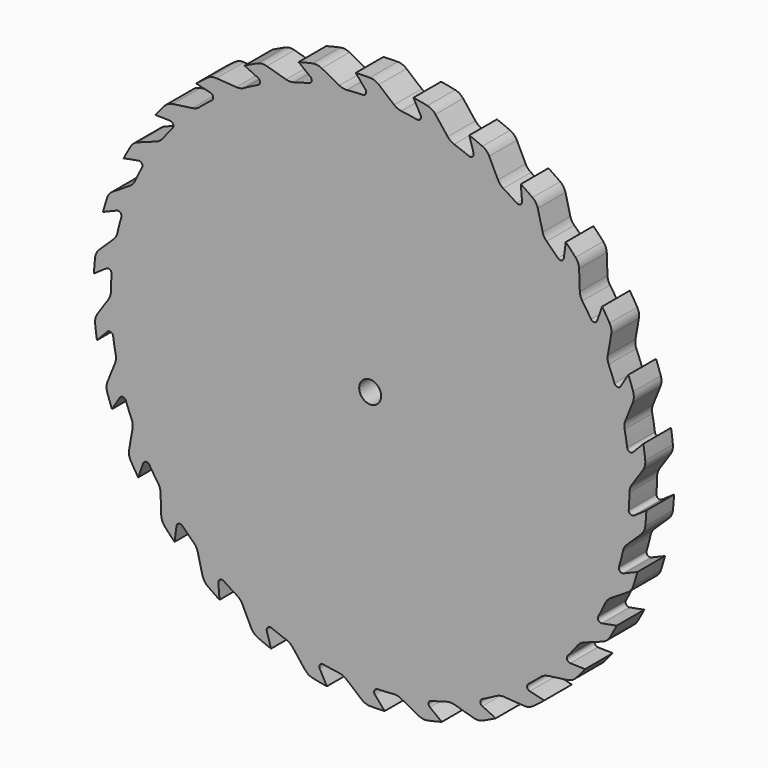
from build123d import *

# Parameters (mm, degrees)
F0_R            = 40
F1_DEPTH        = 5
F4_DEPTH        = 25
F4_COPIES_COUNT = 30
F5_R            = 2
F6_R            = 0.5
F7_R            = 1.5875
F8_DEPTH        = 25


# Not quite as in the source:
# - a pattern or mirror of a feature is missing from the dataset's text; its kind, count and spacing are read off the source's solid


with BuildPart() as f1:
    # F0 (on Front) → F1 (new body)
    with BuildSketch(Plane.XZ):
        Circle(F0_R)
    extrude(amount=F1_DEPTH)

    # F2 (on face) → F4 (cut)
    with BuildSketch(Plane.XZ.offset(5)):
        with BuildLine():
            Line((-7.6323598151, 39.2650873379), (-3.9198173725, 37.2945710763))
            ThreePointArc((-3.9198173725, 37.2945710763), (-1.9625983591, 37.4486075533), (0, 37.5))
            Line((0, 37.5), (-2.0934382497, 39.9451813902))
            ThreePointArc((-2.0934382497, 39.9451813902), (-4.8747737362, 39.7018460657), (-7.6323598151, 39.2650873379))
        make_face()
    f4 = extrude(amount=-F4_DEPTH, mode=Mode.SUBTRACT)

    # F4_copies: F4 ×30 about axis
    f4_copies_axis = Axis((0, 0, 0), (0, 1, 0))
    for i in range(1, F4_COPIES_COUNT):
        add(f4.rotate(f4_copies_axis, i * 360 / F4_COPIES_COUNT), mode=Mode.SUBTRACT)

    # F5
    f5_edges = [f1.edges().sort_by_distance(p)[0] for p in [
        (-7.63236, -2.5, 39.265087),
        (-3.919817, -2.5, 37.294571),
        (0.698096, -2.5, 39.993908),
        (3.919817, -2.5, 37.294571),
        (8.998042, -2.5, 38.974803),
        (11.588137, -2.5, 35.664619),
        (16.90473, -2.5, 36.252311),
        (18.75, -2.5, 32.475953),
        (24.072601, -2.5, 31.94542),
        (25.092398, -2.5, 27.867931),
        (30.188383, -2.5, 26.242361),
        (30.338137, -2.5, 22.041947),
        (34.984788, -2.5, 19.392385),
        (34.257955, -2.5, 15.252624),
        (38.25219, -2.5, 11.694868),
        (36.680535, -2.5, 7.796688),
        (39.847788, -2.5, 3.48623),
        (37.5, -2.5, 0),
        (39.701846, -2.5, -4.874774),
        (36.680535, -2.5, -7.796688),
        (37.820743, -2.5, -13.022726),
        (34.257955, -2.5, -15.252624),
        (34.286692, -2.5, -20.601523),
        (30.338137, -2.5, -22.041947),
        (29.254148, -2.5, -27.279934),
        (25.092398, -2.5, -27.867931),
        (22.943057, -2.5, -32.766082),
        (18.75, -2.5, -32.475953),
        (15.629245, -2.5, -36.820194),
        (11.588137, -2.5, -35.664619),
        (7.63236, -2.5, -39.265087),
        (3.919817, -2.5, -37.294571),
        (-0.698096, -2.5, -39.993908),
        (-3.919817, -2.5, -37.294571),
        (-8.998042, -2.5, -38.974803),
        (-11.588137, -2.5, -35.664619),
        (-16.90473, -2.5, -36.252311),
        (-18.75, -2.5, -32.475953),
        (-24.072601, -2.5, -31.94542),
        (-25.092398, -2.5, -27.867931),
        (-30.188383, -2.5, -26.242361),
        (-30.338137, -2.5, -22.041947),
        (-34.984788, -2.5, -19.392385),
        (-34.257955, -2.5, -15.252624),
        (-38.25219, -2.5, -11.694868),
        (-36.680535, -2.5, -7.796688),
        (-39.847788, -2.5, -3.48623),
        (-37.5, -2.5, 0),
        (-39.701846, -2.5, 4.874774),
        (-36.680535, -2.5, 7.796688),
        (-37.820743, -2.5, 13.022726),
        (-34.257955, -2.5, 15.252624),
        (-34.286692, -2.5, 20.601523),
        (-30.338137, -2.5, 22.041947),
        (-29.254148, -2.5, 27.279934),
        (-25.092398, -2.5, 27.867931),
        (-22.943057, -2.5, 32.766082),
        (-18.75, -2.5, 32.475953),
        (-15.629245, -2.5, 36.820194),
        (-11.588137, -2.5, 35.664619),
    ]]
    fillet(f5_edges, radius=F5_R)

    # F6
    f6_edges = [f1.edges().sort_by_distance(p)[0] for p in [
        (0, -2.5, 37.5),
        (-7.796688, -2.5, 36.680535),
        (7.796688, -2.5, 36.680535),
        (-15.252624, -2.5, 34.257955),
        (15.252624, -2.5, 34.257955),
        (-22.041947, -2.5, 30.338137),
        (22.041947, -2.5, 30.338137),
        (-27.867931, -2.5, 25.092398),
        (27.867931, -2.5, 25.092398),
        (-32.475953, -2.5, 18.75),
        (32.475953, -2.5, 18.75),
        (-35.664619, -2.5, 11.588137),
        (35.664619, -2.5, 11.588137),
        (-37.294571, -2.5, 3.919817),
        (37.294571, -2.5, 3.919817),
        (-37.294571, -2.5, -3.919817),
        (37.294571, -2.5, -3.919817),
        (-35.664619, -2.5, -11.588137),
        (35.664619, -2.5, -11.588137),
        (-32.475953, -2.5, -18.75),
        (32.475953, -2.5, -18.75),
        (-27.867931, -2.5, -25.092398),
        (27.867931, -2.5, -25.092398),
        (-22.041947, -2.5, -30.338137),
        (22.041947, -2.5, -30.338137),
        (-15.252624, -2.5, -34.257955),
        (15.252624, -2.5, -34.257955),
        (-7.796688, -2.5, -36.680535),
        (7.796688, -2.5, -36.680535),
        (0, -2.5, -37.5),
    ]]
    fillet(f6_edges, radius=F6_R)

    # F7 (on face) → F8 (cut)
    with BuildSketch(Plane.XZ.offset(5)):
        Circle(F7_R)
    extrude(amount=-F8_DEPTH, mode=Mode.SUBTRACT)


solid = f1.part
